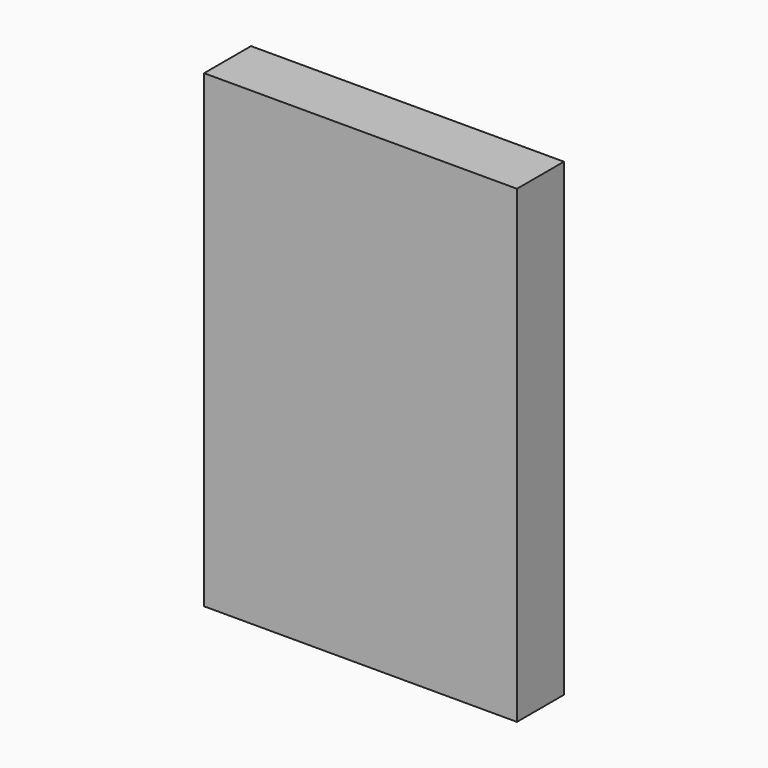
from build123d import *

# Parameters (mm, degrees)
F0_W     = 25.4
F0_H     = 38.1
F1_DEPTH = 4.7625


# Not quite as in the source:
# - a length typed as a fraction of an inch, garbled in the dataset ("3 / 203.2 mm" for 3/8 in), is restored


with BuildPart() as f1:
    # F0 (on Front) → F1 (new body)
    with BuildSketch(Plane.XZ):
        with Locations((12.7, 19.05)):
            Rectangle(F0_W, F0_H)
    extrude(amount=F1_DEPTH)


solid = f1.part
